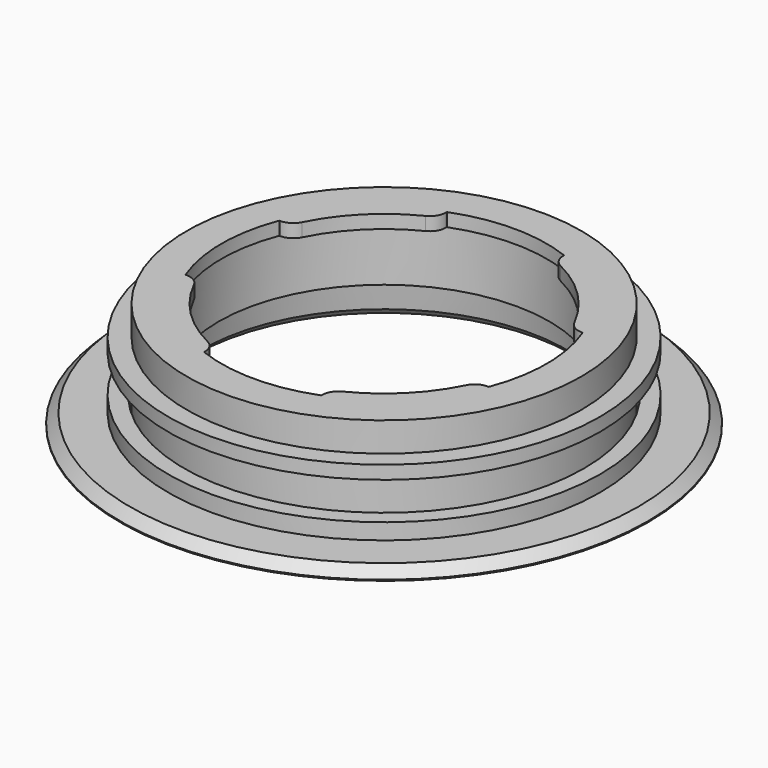
from build123d import *

# Parameters (mm, degrees)
F0_R      = 37
F0_R_2    = 33.5
F1_DEPTH  = 7
F2_R      = 37
F2_R_2    = 33.5
F2_R_3    = 31
F3_DEPTH  = 5
F4_R      = 40.5
F4_R_2    = 37
F4_R_3    = 31
F5_DEPTH  = 2.5
F6_R      = 37
F6_R_2    = 31
F7_DEPTH  = 5.5
F8_R      = 31
F9_DEPTH  = 2.5
F10_SIZE  = 2
F11_R     = 5
F11_R_2   = 1.875
F12_DEPTH = 1.5
F13_R     = 49.5
F13_R_2   = 37.5
F14_DEPTH = 2
F15_R     = 40.5
F15_R_2   = 37.5
F16_DEPTH = 3
F17_SIZE  = 1.8


# Not quite as in the source:
# - a fillet or chamfer that OpenCascade refuses, or shapes differently, is made with other operations: its cross-section is extruded or revolved along the edge and cut away or added


with BuildPart() as f1:
    # F0 (on Top) → F1 (new body)
    with BuildSketch(Plane.XY):
        Circle(F0_R)
        Circle(F0_R_2, mode=Mode.SUBTRACT)
    extrude(amount=F1_DEPTH)

    # F2 (on face) → F3 (join)
    with BuildSketch(Plane.XY.offset(7)):
        Circle(F2_R)
        Circle(F2_R_2, mode=Mode.SUBTRACT)
        Circle(F2_R_2)
        Circle(F2_R_3, mode=Mode.SUBTRACT)
    extrude(amount=F3_DEPTH)

    # F4 (on face) → F5 (join)
    with BuildSketch(Plane.XY.offset(12)):
        Circle(F4_R)
        Circle(F4_R_2, mode=Mode.SUBTRACT)
        Circle(F4_R_2)
        Circle(F4_R_3, mode=Mode.SUBTRACT)
    extrude(amount=F5_DEPTH)

    # F6 (on face) → F7 (join)
    with BuildSketch(Plane.XY.offset(14.5)):
        Circle(F6_R)
        Circle(F6_R_2, mode=Mode.SUBTRACT)
    extrude(amount=F7_DEPTH)

    # F8 (on face) → F9 (join)
    with BuildSketch(Plane.XY.offset(20)):
        Circle(F8_R)
        with BuildLine():
            ThreePointArc((-25.5304828696, 12.6666666667), (-20.1525432638, 20.1525432638), (-12.6666666667, 25.5304828696))
            ThreePointArc((-12.6666666667, 25.5304828696), (-11.4504902432, 26.636763289), (-11, 28.217902119))
            Line((-11, 28.217902119), (-11, 28.4473197331))
            ThreePointArc((-11, 28.4473197331), (0, 30.5), (11, 28.4473197331))
            Line((11, 28.4473197331), (11, 28.217902119))
            ThreePointArc((11, 28.217902119), (11.4504902432, 26.636763289), (12.6666666667, 25.5304828696))
            ThreePointArc((12.6666666667, 25.5304828696), (20.1525432638, 20.1525432638), (25.5304828696, 12.6666666667))
            ThreePointArc((25.5304828696, 12.6666666667), (26.636763289, 11.4504902432), (28.217902119, 11))
            Line((28.217902119, 11), (28.4473197331, 11))
            ThreePointArc((28.4473197331, 11), (30.5, 0), (28.4473197331, -11))
            Line((28.4473197331, -11), (28.217902119, -11))
            ThreePointArc((28.217902119, -11), (26.636763289, -11.4504902432), (25.5304828696, -12.6666666667))
            ThreePointArc((25.5304828696, -12.6666666667), (20.1525432638, -20.1525432638), (12.6666666667, -25.5304828696))
            ThreePointArc((12.6666666667, -25.5304828696), (11.4504902432, -26.636763289), (11, -28.217902119))
            Line((11, -28.217902119), (11, -28.4473197331))
            ThreePointArc((11, -28.4473197331), (0, -30.5), (-11, -28.4473197331))
            Line((-11, -28.4473197331), (-11, -28.217902119))
            ThreePointArc((-11, -28.217902119), (-11.4504902432, -26.636763289), (-12.6666666667, -25.5304828696))
            ThreePointArc((-12.6666666667, -25.5304828696), (-20.1525432638, -20.1525432638), (-25.5304828696, -12.6666666667))
            ThreePointArc((-25.5304828696, -12.6666666667), (-26.636763289, -11.4504902432), (-28.217902119, -11))
            Line((-28.217902119, -11), (-28.4473197331, -11))
            ThreePointArc((-28.4473197331, -11), (-30.5, 0), (-28.4473197331, 11))
            Line((-28.4473197331, 11), (-28.217902119, 11))
            ThreePointArc((-28.217902119, 11), (-26.636763289, 11.4504902432), (-25.5304828696, 12.6666666667))
        make_face(mode=Mode.SUBTRACT)
    extrude(amount=-F9_DEPTH)

    # F10
    f10_edges = [f1.edges().sort_by_distance(p)[0] for p in [
        (-33.5, 0, 0),
    ]]
    chamfer(f10_edges, length=F10_SIZE)

    # F18: chamfer of 5 x 1 on 1 edges, made by hand


with BuildPart() as f12:
    # F11 (on Top) → F12 (new body)
    with BuildSketch(Plane.XY):
        Circle(F11_R)
        Circle(F11_R_2, mode=Mode.SUBTRACT)
    extrude(amount=-F12_DEPTH)


with BuildPart() as f14:
    # F13 (on face) → F14 (new body)
    with BuildSketch(Plane(origin=(0, 0, 0), x_dir=(1, 0, 0), z_dir=(0, 0, -1))):
        Circle(F13_R)
        Circle(F13_R_2, mode=Mode.SUBTRACT)
    extrude(amount=-F14_DEPTH)

    # F15 (on face) → F16 (join)
    with BuildSketch(Plane.XY.offset(2)):
        Circle(F15_R)
        Circle(F15_R_2, mode=Mode.SUBTRACT)
    extrude(amount=F16_DEPTH)

    # F17
    f17_edges = [f14.edges().sort_by_distance(p)[0] for p in [
        (-49.5, 0, 2),
    ]]
    chamfer(f17_edges, length=F17_SIZE)


with BuildPart() as f18_tool2:
    # F18_s3 → F18_t4 (revolve)
    with BuildSketch(Plane.XZ):
        Polygon((34.2071067812, 1.2928932188), (33.5, 7), (33.5, 2), align=None)
    revolve(axis=Axis((0, 0, 2), (0, 0, 1)))

    split(bisect_by=Plane.XY.offset(7), keep=Keep.BOTTOM)


with BuildPart() as f1_1:
    add(f1.part)

    # F18_t1: cut F18_tool2
    add(f18_tool2.part, mode=Mode.SUBTRACT)


solid = Compound([f12.part, f14.part, f1_1.part])
